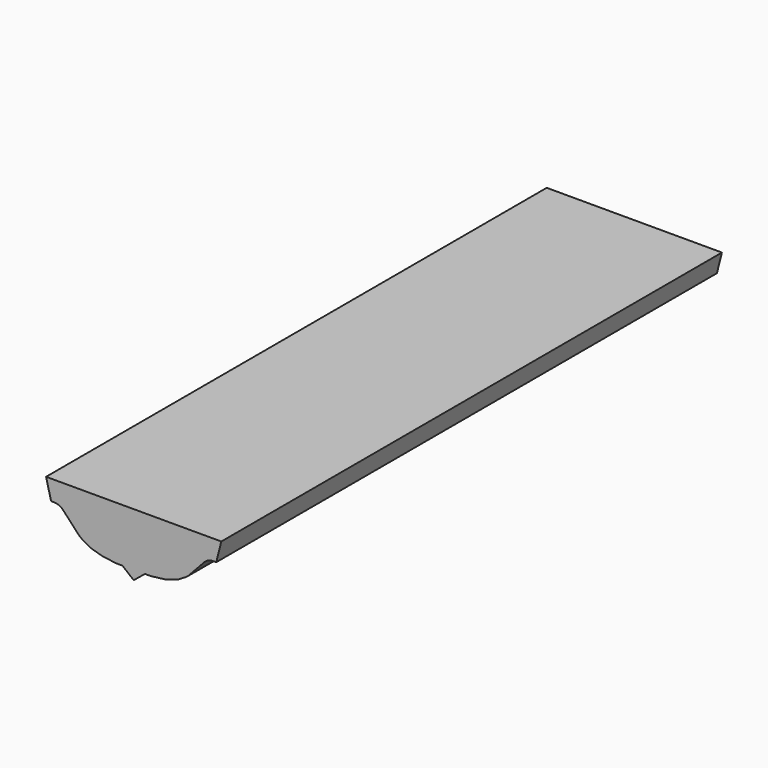
from build123d import *

# Parameters (mm, degrees)
F2_DEPTH = 5000


with BuildPart() as f2:
    # F0 (on Front) → F2 (new body)
    with BuildSketch(Plane.XZ):
        with BuildLine():
            Line((-90.3032645583, 73.3521804214), (0, 0))
            Line((0, 0), (0, 500))
            Line((0, 500), (-700, 500))
            Line((-700, 500), (-659.9707603455, 341.3078779773))
            Line((-659.9707603455, 341.3078779773), (-636.6021653731, 341.3078779773))
            ThreePointArc((-636.6021653731, 341.3078779773), (-596.6712163725, 332.9894972469), (-563.3834841061, 309.4182642155))
            Line((-563.3834841061, 309.4182642155), (-438.5016734996, 175.1702883654))
            ThreePointArc((-438.5016734996, 175.1702883654), (-428.3932790461, 165.710759699), (-417.0752981876, 157.7379540258))
            Line((-417.0752981876, 157.7379540258), (-360.7167568947, 123.615368327))
            ThreePointArc((-360.7167568947, 123.615368327), (-349.2423377723, 117.6459694815), (-337.0934164626, 113.2075319426))
            Line((-337.0934164626, 113.2075319426), (-256.349216299, 89.5028171123))
            ThreePointArc((-256.349216299, 89.5028171123), (-248.5831629557, 87.5568921429), (-240.6863306004, 86.2384660848))
            Line((-240.6863306004, 86.2384660848), (-144.6835198288, 74.1372724315))
            ThreePointArc((-144.6835198288, 74.1372724315), (-138.4427891974, 73.5486464183), (-132.1774400044, 73.3521804214))
            Line((-132.1774400044, 73.3521804214), (-90.3032645583, 73.3521804214))
        make_face()
        with BuildLine():
            Line((0, 500), (0, 0))
            Line((0, 0), (90.3032645583, 73.3521804214))
            Line((90.3032645583, 73.3521804214), (132.1774400044, 73.3521804214))
            ThreePointArc((132.1774400044, 73.3521804214), (138.4427891974, 73.5486464183), (144.6835198288, 74.1372724315))
            Line((144.6835198288, 74.1372724315), (248.6487627029, 87.2421339154))
            Line((248.6487627029, 87.2421339154), (337.0934164626, 113.2075319426))
            ThreePointArc((337.0934164626, 113.2075319426), (349.2423377723, 117.6459694815), (360.7167568947, 123.615368327))
            Line((360.7167568947, 123.615368327), (417.0752981876, 157.7379540258))
            ThreePointArc((417.0752981876, 157.7379540258), (428.3932790461, 165.710759699), (438.5016734996, 175.1702883654))
            Line((438.5016734996, 175.1702883654), (563.3834841061, 309.4182642155))
            ThreePointArc((563.3834841061, 309.4182642155), (596.6712163725, 332.9894972469), (636.6021653731, 341.3078779773))
            Line((636.6021653731, 341.3078779773), (659.9707603455, 341.3078779773))
            Line((659.9707603455, 341.3078779773), (700, 500))
            Line((700, 500), (0, 500))
        make_face()
    extrude(amount=F2_DEPTH)


solid = f2.part
